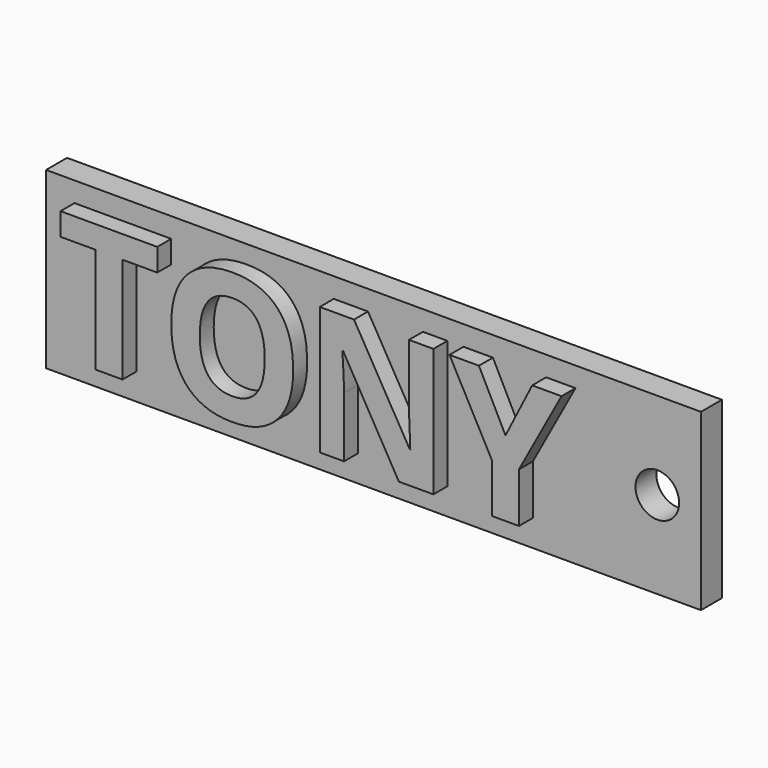
from build123d import *

# Parameters (mm, degrees)
F0_W         = 75
F0_H         = 20
F0_R         = 2.5
F1_DEPTH     = 3
F2_TEXT_SIZE = 20.5473269388
F3_DEPTH     = 2


# Not quite as in the source:
# - Text() gives the source's letters only with a copy of the font that has no kerning and outlines rounded to 1/6400 em; it was checked with that copy


with BuildPart() as f1:
    # F0 (on Front) → F1 (new body)
    with BuildSketch(Plane.XZ):
        with Locations((37.5, -10)):
            Rectangle(F0_W, F0_H)
        with Locations((70, -10)):
            Circle(F0_R, mode=Mode.SUBTRACT)
    extrude(amount=F1_DEPTH)

    # F2 (on face) → F3 (join)
    with BuildSketch(Plane.XZ.offset(3)):
        with Locations((2.8450153768, -16.9562865049)):
            Text('TONY', F2_TEXT_SIZE, font='Open Sans', font_style=FontStyle.BOLD, text_align=(TextAlign.LEFT, TextAlign.BOTTOM))
    extrude(amount=F3_DEPTH)


solid = f1.part
